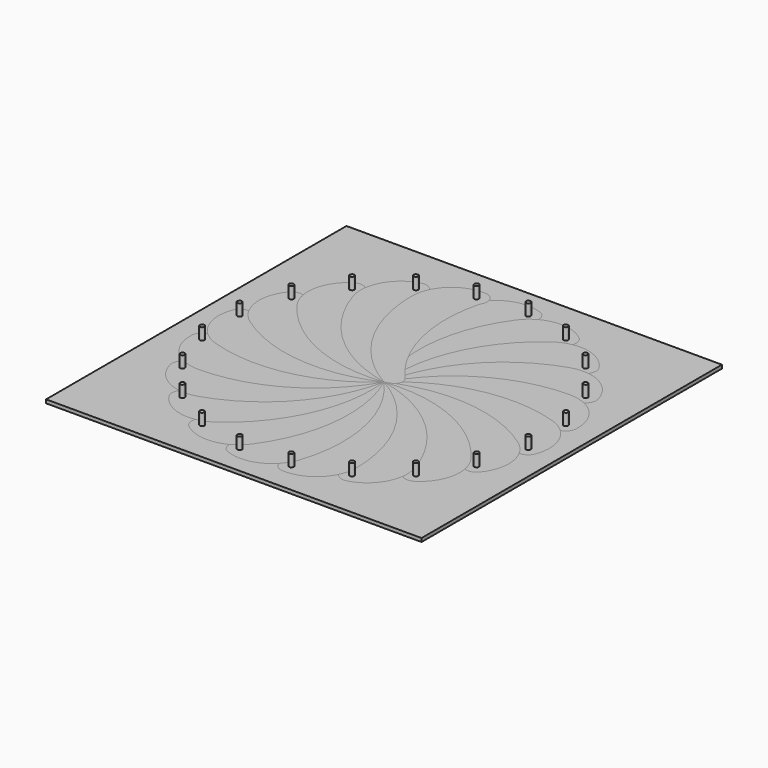
from build123d import *

# Parameters (mm, degrees)
F0_W     = 320
F0_H     = 320
F0_R     = 120
F1_DEPTH = 3
F2_R     = 2
F3_DEPTH = 10
F4_R     = 2
F5_DEPTH = 3
F6_COUNT = 20


# Not quite as in the source:
# - ends of sketch curves that miss each other by under 0.0002 mm in the source are joined


with BuildPart() as f1:
    # F0 (on Top) → F1 (new body)
    with BuildSketch(Plane.XY):
        Rectangle(F0_W, F0_H)
        Circle(F0_R, mode=Mode.SUBTRACT)
    extrude(amount=F1_DEPTH)

    # F2 (on face) → F3 (join)
    with BuildSketch(Plane.XY.offset(3)):
        with Locations((15, 135)):
            Circle(F2_R)
        with Locations((-27.4514464962, 133.0278846155)):
            Circle(F2_R)
        with Locations((-67.2157541439, 118.034073025)):
            Circle(F2_R)
        with Locations((-100.4005154562, 91.4862639751)):
            Circle(F2_R)
        with Locations((-123.7573747842, 55.983141985)):
            Circle(F2_R)
        with Locations((-135, 15)):
            Circle(F2_R)
        with Locations((-133.0278846155, -27.4514464962)):
            Circle(F2_R)
        with Locations((-118.034073025, -67.2157541439)):
            Circle(F2_R)
        with Locations((-91.4862639751, -100.4005154562)):
            Circle(F2_R)
        with Locations((-55.983141985, -123.7573747842)):
            Circle(F2_R)
        with Locations((-15, -135)):
            Circle(F2_R)
        with Locations((27.4514464962, -133.0278846155)):
            Circle(F2_R)
        with Locations((67.2157541439, -118.034073025)):
            Circle(F2_R)
        with Locations((100.4005154562, -91.4862639751)):
            Circle(F2_R)
        with Locations((123.7573747842, -55.983141985)):
            Circle(F2_R)
        with Locations((135, -15)):
            Circle(F2_R)
        with Locations((133.0278846155, 27.4514464962)):
            Circle(F2_R)
        with Locations((118.034073025, 67.2157541439)):
            Circle(F2_R)
        with Locations((91.4862639751, 100.4005154562)):
            Circle(F2_R)
        with Locations((55.983141985, 123.7573747842)):
            Circle(F2_R)
    extrude(amount=F3_DEPTH)


with BuildPart() as f5:
    # F4 (on Top) → F5 (new body)
    with BuildSketch(Plane.XY):
        with BuildLine():
            ThreePointArc((18.3028030826, 143.3720661606), (-8.7043851765, 142.4754508959), (-26.5166067859, 122.1550941586))
            ThreePointArc((-26.5166067859, 122.1550941586), (-26.523252159, 122.1343975098), (-26.5298746493, 122.1136935159))
            ThreePointArc((-26.5298746493, 122.1136935159), (-29.6193802213, 57.503753673), (0, 0))
            Line((0, 0), (4.7717340097, 0))
            ThreePointArc((4.7717340097, 0), (10.6379363494, 3.1806191457), (11.1732371251, 9.8320942541))
            ThreePointArc((11.1732371251, 9.8320942541), (0.8397813845, 69.8058361879), (20.0514591299, 127.5513249058))
            ThreePointArc((20.0514591299, 127.5513249058), (23.9455233353, 135.9887427665), (18.3028030826, 143.3720661606))
        make_face()
        with Locations((15, 135)):
            Circle(F4_R, mode=Mode.SUBTRACT)
    extrude(amount=F5_DEPTH)


with BuildPart() as f6_1:
    # F6: instance of F5
    add(f5.part.rotate(Axis((0, 0, 3), (0, 0, -1)), 1 * 360 / F6_COUNT))


with BuildPart() as f6_2:
    # F6: instance of F5
    add(f5.part.rotate(Axis((0, 0, 3), (0, 0, -1)), 2 * 360 / F6_COUNT))


with BuildPart() as f6_3:
    # F6: instance of F5
    add(f5.part.rotate(Axis((0, 0, 3), (0, 0, -1)), 3 * 360 / F6_COUNT))


with BuildPart() as f6_4:
    # F6: instance of F5
    add(f5.part.rotate(Axis((0, 0, 3), (0, 0, -1)), 4 * 360 / F6_COUNT))


with BuildPart() as f6_5:
    # F6: instance of F5
    add(f5.part.rotate(Axis((0, 0, 3), (0, 0, -1)), 5 * 360 / F6_COUNT))


with BuildPart() as f6_6:
    # F6: instance of F5
    add(f5.part.rotate(Axis((0, 0, 3), (0, 0, -1)), 6 * 360 / F6_COUNT))


with BuildPart() as f6_7:
    # F6: instance of F5
    add(f5.part.rotate(Axis((0, 0, 3), (0, 0, -1)), 7 * 360 / F6_COUNT))


with BuildPart() as f6_8:
    # F6: instance of F5
    add(f5.part.rotate(Axis((0, 0, 3), (0, 0, -1)), 8 * 360 / F6_COUNT))


with BuildPart() as f6_9:
    # F6: instance of F5
    add(f5.part.rotate(Axis((0, 0, 3), (0, 0, -1)), 9 * 360 / F6_COUNT))


with BuildPart() as f6_10:
    # F6: instance of F5
    add(f5.part.rotate(Axis((0, 0, 3), (0, 0, -1)), 10 * 360 / F6_COUNT))


with BuildPart() as f6_11:
    # F6: instance of F5
    add(f5.part.rotate(Axis((0, 0, 3), (0, 0, -1)), 11 * 360 / F6_COUNT))


with BuildPart() as f6_12:
    # F6: instance of F5
    add(f5.part.rotate(Axis((0, 0, 3), (0, 0, -1)), 12 * 360 / F6_COUNT))


with BuildPart() as f6_13:
    # F6: instance of F5
    add(f5.part.rotate(Axis((0, 0, 3), (0, 0, -1)), 13 * 360 / F6_COUNT))


with BuildPart() as f6_14:
    # F6: instance of F5
    add(f5.part.rotate(Axis((0, 0, 3), (0, 0, -1)), 14 * 360 / F6_COUNT))


with BuildPart() as f6_15:
    # F6: instance of F5
    add(f5.part.rotate(Axis((0, 0, 3), (0, 0, -1)), 15 * 360 / F6_COUNT))


with BuildPart() as f6_16:
    # F6: instance of F5
    add(f5.part.rotate(Axis((0, 0, 3), (0, 0, -1)), 16 * 360 / F6_COUNT))


with BuildPart() as f6_17:
    # F6: instance of F5
    add(f5.part.rotate(Axis((0, 0, 3), (0, 0, -1)), 17 * 360 / F6_COUNT))


with BuildPart() as f6_18:
    # F6: instance of F5
    add(f5.part.rotate(Axis((0, 0, 3), (0, 0, -1)), 18 * 360 / F6_COUNT))


with BuildPart() as f6_19:
    # F6: instance of F5
    add(f5.part.rotate(Axis((0, 0, 3), (0, 0, -1)), 19 * 360 / F6_COUNT))


solid = Compound([f1.part, f5.part, f6_1.part, f6_2.part, f6_3.part, f6_4.part, f6_5.part, f6_6.part, f6_7.part, f6_8.part, f6_9.part, f6_10.part, f6_11.part, f6_12.part, f6_13.part, f6_14.part, f6_15.part, f6_16.part, f6_17.part, f6_18.part, f6_19.part])
